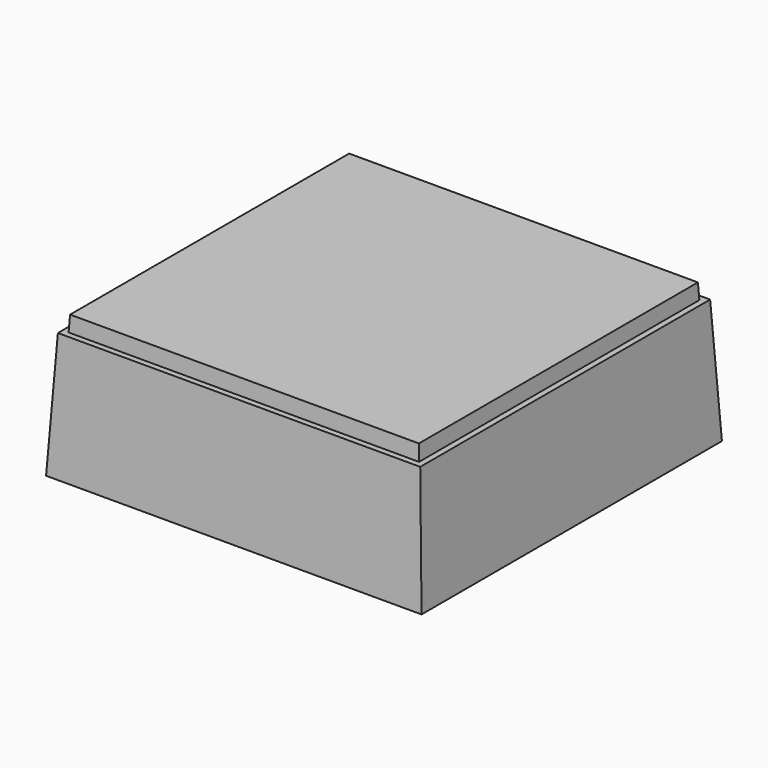
from build123d import *

# Parameters (mm, degrees)
F0_W     = 38.1
F0_H     = 38.1
F1_DEPTH = 25.4
F1_TAPER = 3
F2_W     = 71.12
F2_H     = 71.12
F3_DEPTH = 3.175
F3_TAPER = 3


# Not quite as in the source:
# - a feature of the source that left no trace in its solid (it failed there, or was rolled back) is left out


with BuildPart() as f1:
    # F0 (on Top) → F1 (new body)
    with BuildSketch(Plane.XY):
        with Locations((-19.05, 19.05)):
            Rectangle(F0_W, F0_H)
        with Locations((19.05, 19.05)):
            Rectangle(F0_W, F0_H)
        with Locations((-19.05, -19.05)):
            Rectangle(F0_W, F0_H)
        with Locations((19.05, -19.05)):
            Rectangle(F0_W, F0_H)
    extrude(amount=F1_DEPTH, taper=F1_TAPER)

    # F2 (on face) → F3 (join)
    with BuildSketch(Plane.XY.offset(25.4)):
        Rectangle(F2_W, F2_H)
    extrude(amount=F3_DEPTH, taper=F3_TAPER)


solid = f1.part
